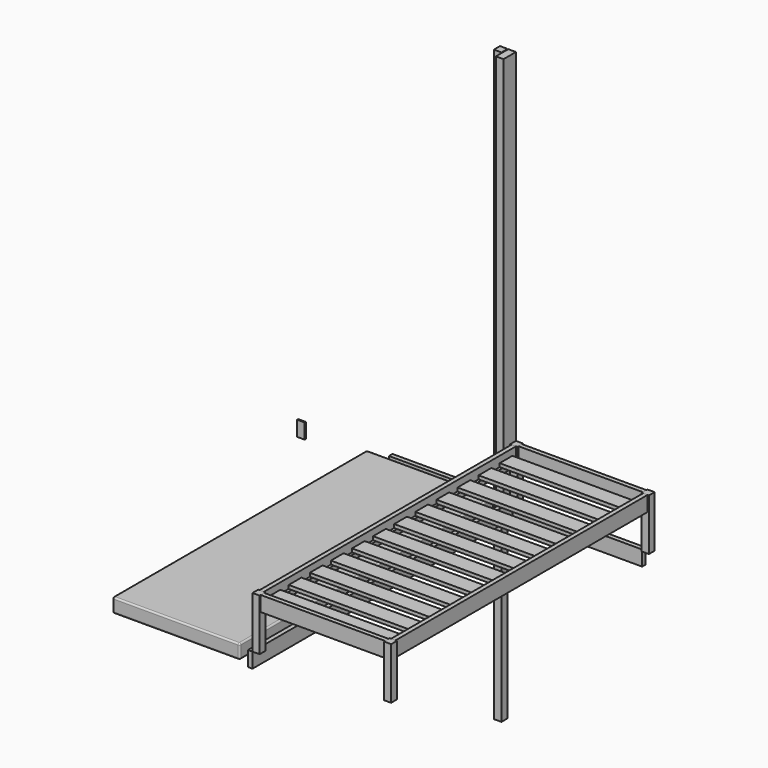
from build123d import *

# Parameters (mm, degrees)
F0_W      = 45
F0_H      = 45
F1_DEPTH  = 320
F5_W      = 28
F5_H      = 95
F6_DEPTH  = 2000
F14_W     = 28
F14_H     = 90
F15_DEPTH = 1983
F18_W     = 28
F18_H     = 90
F19_DEPTH = 783
F22_W     = 18
F22_H     = 32
F23_DEPTH = 1963
F26_W     = 100
F26_H     = 22
F27_DEPTH = 800
F55_DEPTH = 5
F56_DEPTH = 5
F57_DEPTH = 5
F58_DEPTH = 5
F59_DEPTH = 5
F60_DEPTH = 5
F61_DEPTH = 5
F62_DEPTH = 5
F63_W     = 48
F63_H     = 98
F64_DEPTH = 2480
F65_W     = 48
F65_H     = 48
F66_DEPTH = 2480
F68_W     = 28
F68_H     = 95
F69_DEPTH = 817
F67_W     = 28
F67_H     = 95
F70_DEPTH = 2073
F71_W     = 800
F71_H     = 90
F72_DEPTH = 2000
F73_R     = 10
F74_DEPTH = 1230
F75_DEPTH = 777
F76_DEPTH = 364.5
F77_W     = 48
F77_H     = 95
F78_DEPTH = 8.5
F79_DEPTH = 432.5


with BuildPart() as f1:
    # F0 (on Top) → F1 (new body)
    with BuildSketch(Plane.XY):
        with Locations((22.5, -22.5)):
            Rectangle(F0_W, F0_H)
    extrude(amount=F1_DEPTH)


with BuildPart() as f2_1:
    # F2: copy of F1
    add(f1.part.moved(Location((845, 0, 0))))


with BuildPart() as f3_1:
    # F3: copy of F1
    add(f1.part.moved(Location((0, -2045, 0))))


with BuildPart() as f4_1:
    # F4: copy of F2_1
    add(f2_1.part.moved(Location((0, -2045, 0))))


with BuildPart() as f6:
    # F5 (on face) → F6 (new body)
    with BuildSketch(Plane.XZ.offset(45)):
        with Locations((14, 272.5)):
            Rectangle(F5_W, F5_H)
    extrude(amount=F6_DEPTH)


with BuildPart() as f6_1:
    # F7: moved
    add(f6.part.moved(Location((8.5, 0, 0))))


with BuildPart() as f8_1:
    # F8: copy of F6
    add(f6_1.part.moved(Location((828, 0, 0))))


with BuildPart() as f2_1_1:
    # F9: moved
    add(f2_1.part.moved(Location((-17, 0, 0))))

    # F62 (add): a face of the model
    f62_faces = [f2_1_1.faces().sort_by_distance(p)[0] for p in [
        (850.5, -22.5, 320),
    ]]
    extrude(f62_faces, amount=F62_DEPTH)


with BuildPart() as f4_1_1:
    # F10: moved
    add(f4_1.part.moved(Location((-17, 0, 0))))


with BuildPart() as f3_1_1:
    # F12: moved
    add(f3_1.part.moved(Location((0, 17, 0))))

    # F60 (add): a face of the model
    f60_faces = [f3_1_1.faces().sort_by_distance(p)[0] for p in [
        (22.5, -2050.5, 320),
    ]]
    extrude(f60_faces, amount=F60_DEPTH)


with BuildPart() as f4_1_2:
    # F13: moved
    add(f4_1_1.part.moved(Location((0, 17, 0))))

    # F59 (add): a face of the model
    f59_faces = [f4_1_2.faces().sort_by_distance(p)[0] for p in [
        (850.5, -2050.5, 320),
    ]]
    extrude(f59_faces, amount=F59_DEPTH)


with BuildPart() as f15:
    # F14 (on face) → F15 (new body)
    with BuildSketch(Plane.XZ.offset(45)):
        with Locations((14, 275)):
            Rectangle(F14_W, F14_H)
    extrude(amount=F15_DEPTH)


with BuildPart() as f15_1:
    # F16: moved
    add(f15.part.moved(Location((8.5, 0, 0))))


with BuildPart() as f17_1:
    # F17: copy of F15
    add(f15_1.part.moved(Location((828, 0, 0))))

    # F55 (add): a face of the model
    f55_faces = [f17_1.faces().sort_by_distance(p)[0] for p in [
        (850.5, -1036.5, 320),
    ]]
    extrude(f55_faces, amount=F55_DEPTH)


with BuildPart() as f19:
    # F18 (on face) → F19 (new body)
    with BuildSketch(Plane.YZ.offset(45)):
        with Locations((-14, 275)):
            Rectangle(F18_W, F18_H)
    extrude(amount=F19_DEPTH)


with BuildPart() as f19_1:
    # F20: moved
    add(f19.part.moved(Location((0, -8.5, 0))))


with BuildPart() as f21_1:
    # F21: copy of F19
    add(f19_1.part.moved(Location((0, -2028, 0))))

    # F57 (add): a face of the model
    f57_faces = [f21_1.faces().sort_by_distance(p)[0] for p in [
        (436.5, -2050.5, 320),
    ]]
    extrude(f57_faces, amount=F57_DEPTH)


with BuildPart() as f23:
    # F22 (on face) → F23 (new body)
    with BuildSketch(Plane.XZ.offset(45)):
        with Locations((36, 304)):
            Rectangle(F22_W, F22_H)
    extrude(amount=F23_DEPTH)


with BuildPart() as f23_1:
    # F24: moved
    add(f23.part.moved(Location((9.5, -10, -58))))


with BuildPart() as f25_1:
    # F25: copy of F23
    add(f23_1.part.moved(Location((782, 0, 0))))


with BuildPart() as f27:
    # F26 (on face) → F27 (new body)
    with BuildSketch(Plane.YZ.offset(54.5)):
        with Locations((-105, 273)):
            Rectangle(F26_W, F26_H)
    extrude(amount=F27_DEPTH)


with BuildPart() as f27_1:
    # F28: moved
    add(f27.part.moved(Location((-18, 0, 0))))


with BuildPart() as f27_2:
    # F29: moved
    add(f27_1.part.moved(Location((0, -21.5, 0))))


with BuildPart() as f30_1:
    # F30: copy of F27
    add(f27_2.part.moved(Location((0, -160, 0))))


with BuildPart() as f30_1_1:
    # F31: moved
    add(f30_1.part.moved(Location((0, -160, 0))))


with BuildPart() as f32_1:
    # F32: copy of F27
    add(f27_2.part.moved(Location((0, -160, 0))))


with BuildPart() as f33_1:
    # F33: copy of F30_1
    add(f30_1_1.part.moved(Location((0, -160, 0))))


with BuildPart() as f34_1:
    # F34: copy of F33_1
    add(f33_1.part.moved(Location((0, -160, 0))))


with BuildPart() as f35_1:
    # F35: copy of F34_1
    add(f34_1.part.moved(Location((0, -160, 0))))


with BuildPart() as f36_1:
    # F36: copy of F35_1
    add(f35_1.part.moved(Location((0, -160, 0))))


with BuildPart() as f37_1:
    # F37: copy of F36_1
    add(f36_1.part.moved(Location((0, -160, 0))))


with BuildPart() as f38_1:
    # F38: copy of F37_1
    add(f37_1.part.moved(Location((0, -160, 0))))


with BuildPart() as f39_1:
    # F39: copy of F38_1
    add(f38_1.part.moved(Location((0, -160, 0))))


with BuildPart() as f40_1:
    # F40: copy of F39_1
    add(f39_1.part.moved(Location((0, -160, 0))))


with BuildPart() as f41_1:
    # F41: copy of F40_1
    add(f40_1.part.moved(Location((0, -160, 0))))


with BuildPart() as f27_3:
    # F43: moved
    add(f27_2.part.moved(Location((0, 3, 0))))


with BuildPart() as f44_1:
    # F44: copy of F27
    add(f27_3.part.moved(Location((0, -166, 0))))


with BuildPart() as f45_1:
    # F45: copy of F44_1
    add(f44_1.part.moved(Location((0, -166, 0))))


with BuildPart() as f46_1:
    # F46: copy of F45_1
    add(f45_1.part.moved(Location((0, -166, 0))))


with BuildPart() as f47_1:
    # F47: copy of F46_1
    add(f46_1.part.moved(Location((0, -166, 0))))


with BuildPart() as f48_1:
    # F48: copy of F47_1
    add(f47_1.part.moved(Location((0, -166, 0))))


with BuildPart() as f49_1:
    # F49: copy of F48_1
    add(f48_1.part.moved(Location((0, -166, 0))))


with BuildPart() as f50_1:
    # F50: copy of F49_1
    add(f49_1.part.moved(Location((0, -166, 0))))


with BuildPart() as f51_1:
    # F51: copy of F50_1
    add(f50_1.part.moved(Location((0, -166, 0))))


with BuildPart() as f52_1:
    # F52: copy of F51_1
    add(f51_1.part.moved(Location((0, -166, 0))))


with BuildPart() as f53_1:
    # F53: copy of F52_1
    add(f52_1.part.moved(Location((0, -166, 0))))


with BuildPart() as f54_1:
    # F54: copy of F53_1
    add(f53_1.part.moved(Location((0, -166, 0))))


with BuildPart() as f19_2:
    add(f19_1.part)

    # F56 (add): a face of the model
    f56_faces = [f19_2.faces().sort_by_distance(p)[0] for p in [
        (436.5, -22.5, 320),
    ]]
    extrude(f56_faces, amount=F56_DEPTH)


with BuildPart() as f15_2:
    add(f15_1.part)

    # F58 (add): a face of the model
    f58_faces = [f15_2.faces().sort_by_distance(p)[0] for p in [
        (22.5, -1036.5, 320),
    ]]
    extrude(f58_faces, amount=F58_DEPTH)


with BuildPart() as f1_1:
    add(f1.part)

    # F61 (add): a face of the model
    f61_faces = [f1_1.faces().sort_by_distance(p)[0] for p in [
        (22.5, -22.5, 320),
    ]]
    extrude(f61_faces, amount=F61_DEPTH)


with BuildPart() as f64:
    # F63 (on Top) → F64 (new body)
    with BuildSketch(Plane.XY):
        with Locations((-24, -49)):
            Rectangle(F63_W, F63_H)
    extrude(amount=F64_DEPTH)


with BuildPart() as f66:
    # F65 (on Top) → F66 (new body)
    with BuildSketch(Plane.XY):
        with Locations((-76.6017923355, -24)):
            Rectangle(F65_W, F65_H)
    extrude(amount=F66_DEPTH)


with BuildPart() as f69:
    # F68 (on Right) → F69 (new body)
    with BuildSketch(Plane.YZ):
        with Locations((-14, -47.5)):
            Rectangle(F68_W, F68_H)
    extrude(amount=F69_DEPTH)


with BuildPart() as f70:
    # F67 (on Front) → F70 (new body)
    with BuildSketch(Plane.XZ):
        with Locations((-14, -47.5)):
            Rectangle(F67_W, F67_H)
    extrude(amount=F70_DEPTH)


with BuildPart() as f72:
    # F71 (on face) → F72 (new body)
    with BuildSketch(Plane.XZ.offset(48)):
        with Locations((-500.6017923355, -45)):
            Rectangle(F71_W, F71_H)
    extrude(amount=F72_DEPTH)

    # F73
    f73_edges = [f72.edges().sort_by_distance(p)[0] for p in [
        (-900.601792, -1048, 0),
        (-900.601792, -1048, -90),
        (-900.601792, -48, -45),
        (-500.601792, -48, 0),
        (-500.601792, -48, -90),
        (-900.601792, -2048, -45),
        (-500.601792, -2048, 0),
        (-500.601792, -2048, -90),
        (-100.601792, -2048, -45),
        (-100.601792, -1048, 0),
        (-100.601792, -1048, -90),
        (-100.601792, -48, -45),
    ]]
    fillet(f73_edges, radius=F73_R)


with BuildPart() as f74:
    # F65 (on Top) → F74 (new body)
    with BuildSketch(Plane.XY):
        with Locations((-76.6017923355, -24)):
            Rectangle(F65_W, F65_H)
    extrude(amount=-F74_DEPTH)


with BuildPart() as f75:
    # F68 (on Right) → F75 (new body)
    with BuildSketch(Plane.YZ):
        with Locations((-14, -47.5)):
            Rectangle(F68_W, F68_H)
    extrude(amount=-F75_DEPTH)


with BuildPart() as f76:
    # F68 (on Right) → F76 (new body)
    with BuildSketch(Plane.YZ):
        with Locations((-14, -47.5)):
            Rectangle(F68_W, F68_H)
    extrude(amount=-F76_DEPTH)


with BuildPart() as f78:
    # F77 (on Front) → F78 (new body)
    with BuildSketch(Plane.XZ):
        with Locations((-1346.6387281418, -47.5)):
            Rectangle(F77_W, F77_H)
    extrude(amount=F78_DEPTH)


with BuildPart() as f79:
    # F68 (on Right) → F79 (new body)
    with BuildSketch(Plane.YZ):
        with Locations((-14, -47.5)):
            Rectangle(F68_W, F68_H)
    extrude(amount=-F79_DEPTH)


solid = Compound([f2_1_1.part, f3_1_1.part, f4_1_2.part, f17_1.part, f21_1.part, f23_1.part, f25_1.part, f27_3.part, f44_1.part, f45_1.part, f46_1.part, f47_1.part, f48_1.part, f49_1.part, f50_1.part, f51_1.part, f52_1.part, f53_1.part, f54_1.part, f19_2.part, f15_2.part, f1_1.part, f64.part, f66.part, f69.part, f70.part, f72.part, f74.part, f75.part, f76.part, f78.part, f79.part])
